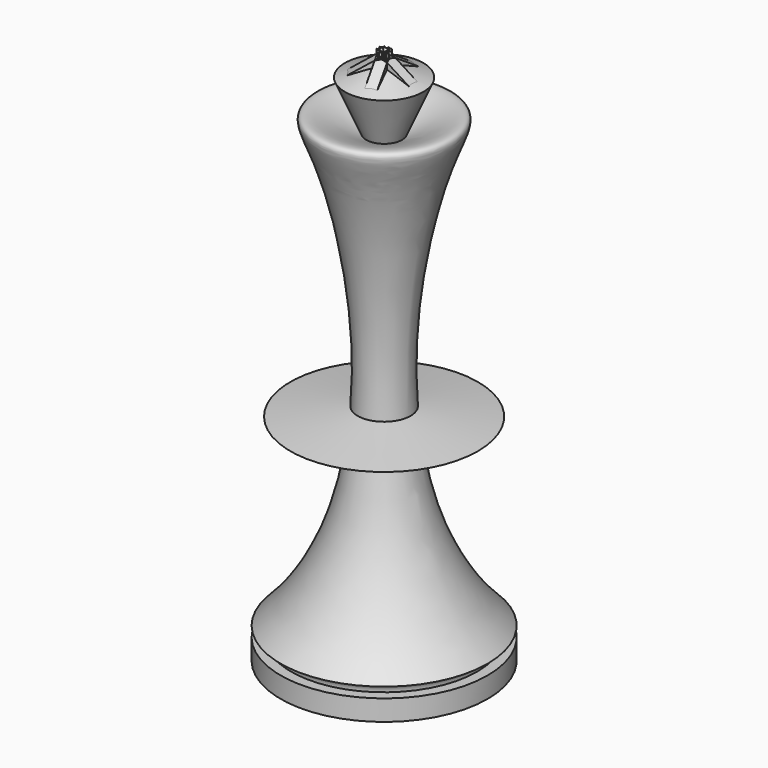
from build123d import *

# Parameters (mm, degrees)
F3_DEPTH = 0.5
F4_COUNT = 5


# Not quite as in the source:
# - a feature names something its author has since deleted; it is built from what else it names


with BuildPart() as f1:
    # F0 (on Front) → F1 (revolve)
    with BuildSketch(Plane.XZ):
        with BuildLine():
            Line((0, 9.0353097767), (0, 0))
            Line((0, 0), (10, 0))
            Line((10, 0), (10, 2))
            Line((10, 2), (9, 2))
            ThreePointArc((9, 2), (9.2928932188, 2.7071067812), (10, 3))
            add(Edge.make_bspline(
                [(10, 3), (5.8599692942, 7.1514955665), (3.7520111059, 12.6606088045), (2.9057694535, 18.3767723616)],
                knots=[0, 0, 0, 0, 0.2723692437, 0.2723692437, 0.2723692437, 0.2723692437], degree=3))
            Line((2.9057694535, 18.3767723616), (1.4480197044, 17.810525763))
            Line((1.4480197044, 17.810525763), (2.4403755087, 11.1617380753))
            Line((2.4403755087, 11.1617380753), (0, 9.0353097767))
        make_face()
        with BuildLine():
            Line((0, 51), (0, 44))
            add(Edge.make_bspline(
                [(1.7302031744, 44.8584092014), (1.2074659957, 44.6052050311), (0.6322180551, 44.3196864642), (0, 44)],
                knots=[0.9786462718, 0.9786462718, 0.9786462718, 0.9786462718, 1, 1, 1, 1], degree=3))
            Line((1.7302031744, 44.8584092014), (3.7866074126, 49.6094115078))
            Line((3.7866074126, 49.6094115078), (0, 51))
        make_face()
        with BuildLine():
            Line((1.1113585206, 20.0661569834), (1.4480197044, 17.810525763))
            Line((1.4480197044, 17.810525763), (2.9057694535, 18.3767723616))
            add(Edge.make_bspline(
                [(2.9057694535, 18.3767723616), (2.7448272283, 19.4638992829), (2.6295215739, 20.5585152608), (2.554553193, 21.6527055151)],
                knots=[0.2723692437, 0.2723692437, 0.2723692437, 0.2723692437, 0.32416971, 0.32416971, 0.32416971, 0.32416971], degree=3))
            Line((2.554553193, 21.6527055151), (1.1113585206, 21.8489095134))
            Line((1.1113585206, 21.8489095134), (1.1113585206, 20.0661569834))
        make_face()
        with BuildLine():
            add(Edge.make_bspline(
                [(2.9057694535, 18.3767723616), (2.7448272283, 19.4638992829), (2.6295215739, 20.5585152608), (2.554553193, 21.6527055151)],
                knots=[0.2723692437, 0.2723692437, 0.2723692437, 0.2723692437, 0.32416971, 0.32416971, 0.32416971, 0.32416971], degree=3))
            Line((2.9057694535, 18.3767723616), (9.0618459508, 20.7680314779))
            Line((9.0618459508, 20.7680314779), (2.554553193, 21.6527055151))
        make_face()
        with BuildLine():
            Line((0, 44), (0, 41.3304418325))
            Line((0, 41.3304418325), (2.4403755087, 41.3304418325))
            Line((2.4403755087, 41.3304418325), (1.1113585206, 31.4957089722))
            Line((1.1113585206, 31.4957089722), (1.1113585206, 21.8489095134))
            Line((1.1113585206, 21.8489095134), (2.554553193, 21.6527055151))
            add(Edge.make_bspline(
                [(2.554553193, 21.6527055151), (1.9701230673, 30.1826716243), (4.9959561324, 43.9653621083), (7.8662442935, 47.8305934345), (1.7302031744, 44.8584092014)],
                knots=[0.32416971, 0.32416971, 0.32416971, 0.32416971, 0.727989996, 0.9786462718, 0.9786462718, 0.9786462718, 0.9786462718], degree=3))
            add(Edge.make_bspline(
                [(1.7302031744, 44.8584092014), (1.2074659957, 44.6052050311), (0.6322180551, 44.3196864642), (0, 44)],
                knots=[0.9786462718, 0.9786462718, 0.9786462718, 0.9786462718, 1, 1, 1, 1], degree=3))
        make_face()
    revolve(axis=Axis((0, 0, 22), (0, 0, 1)))



with BuildPart() as f3:
    # F2 (on Front) → F3 (new body, symmetric)
    with BuildSketch(Plane.XZ):
        Polygon((-0.3592191799, 51.9545889315), (-0.3592191799, 50.8362587973), (3.4741000272, 49.5302081108), align=None)
    extrude(amount=F3_DEPTH, both=True)


with BuildPart() as f1_1:
    add(f1.part)

    add(f3.part)  # F4 merges F3
    # F4: F3 ×5 about axis
    f4_axis = Axis((0, 0, 47.5), (0, 0, 1))
    for i in range(1, F4_COUNT):
        add(f3.part.rotate(f4_axis, i * 360 / F4_COUNT))


solid = f1_1.part
